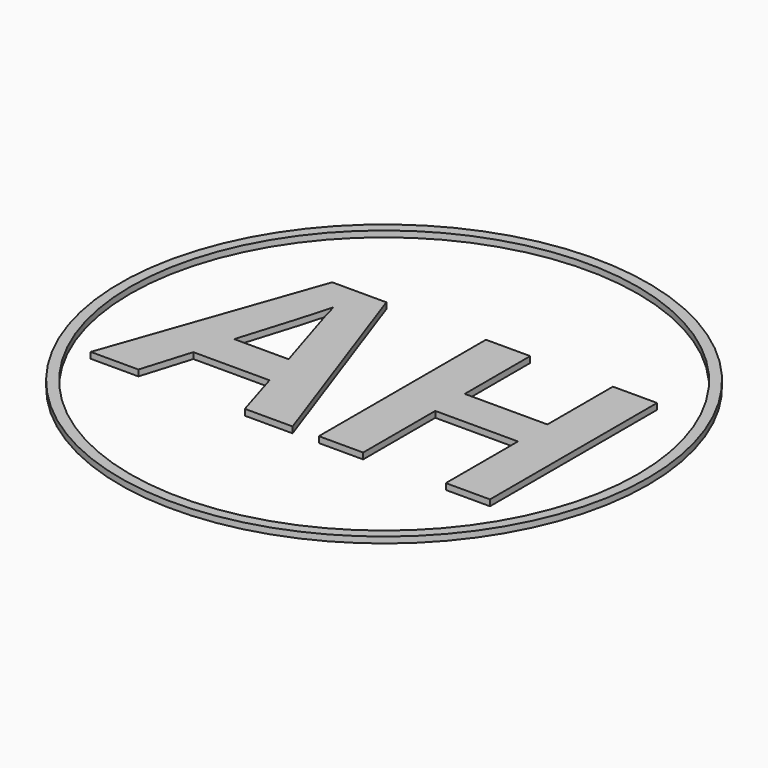
from build123d import *

# Parameters (mm, degrees)
F1_TEXT_SIZE = 18.2991038251
F2_R         = 16.51
F2_R_2       = 15.875
F3_DEPTH     = 0.381


# Not quite as in the source:
# - Text() gives the source's letters only with a copy of the font that has no kerning and outlines rounded to 1/6400 em; it was checked with that copy


with BuildPart() as f3:
    # F1 (on offset) + F2 (on offset) → F3 (new body)
    with BuildSketch(Plane.XY.offset(3.302)):
        with Locations((-13.081, -6.587677377)):
            Text('AH', F1_TEXT_SIZE, font='Open Sans', font_style=FontStyle.BOLD, text_align=(TextAlign.LEFT, TextAlign.BOTTOM))
    with BuildSketch(Plane.XY.offset(3.302)):
        Circle(F2_R)
        Circle(F2_R_2, mode=Mode.SUBTRACT)
    extrude(amount=-F3_DEPTH)


solid = f3.part
